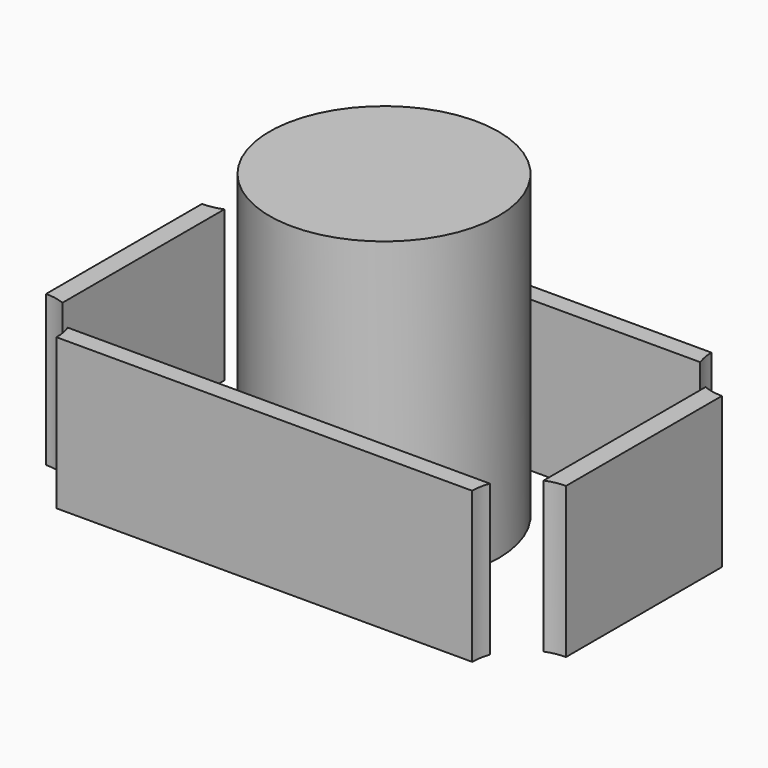
from build123d import *

# Parameters (mm, degrees)
F1_DEPTH = 25.4
F0_R     = 19.2971097636
F3_DEPTH = 50.8


# Not quite as in the source:
# - the program builds the solid bodies; features that only make, move or delete a surface that nothing else refers to are left out


with BuildPart() as f1:
    # F0 (on Top) → F1 (new body)
    with BuildSketch(Plane.XY):
        with BuildLine():
            Line((35.0388884567, 25.2227913588), (-35.0388884567, 25.2227913588))
            ThreePointArc((-35.0388884567, 25.2227913588), (-35.1771760377, 23.6696604158), (-35.5876880321, 22.1653934568))
            Line((-35.5876880321, 22.1653934568), (35.5876880321, 22.1653934568))
            ThreePointArc((35.5876880321, 22.1653934568), (35.1771760377, 23.6696604158), (35.0388884567, 25.2227913588))
        make_face()
    extrude(amount=F1_DEPTH)


with BuildPart() as f1b:
    # F0 (on Top) → F1, piece 2 (new body)
    with BuildSketch(Plane.XY):
        with BuildLine():
            Line((40.5652746558, 17.0605210708), (40.5652746558, -17.0605210708))
            ThreePointArc((40.5652746558, -17.0605210708), (42.1675359576, -16.590493834), (43.8297688961, -16.4319109195))
            Line((43.8297688961, -16.4319109195), (43.8297688961, 16.4319109195))
            ThreePointArc((43.8297688961, 16.4319109195), (42.1675359576, 16.590493834), (40.5652746558, 17.0605210708))
        make_face()
    extrude(amount=F1_DEPTH)


with BuildPart() as f1c:
    # F0 (on Top) → F1, piece 3 (new body)
    with BuildSketch(Plane.XY):
        with BuildLine():
            Line((-43.8297688961, 16.4319109195), (-43.8297688961, -16.4319109195))
            ThreePointArc((-43.8297688961, -16.4319109195), (-42.1675359576, -16.590493834), (-40.5652746558, -17.0605210708))
            Line((-40.5652746558, -17.0605210708), (-40.5652746558, 17.0605210708))
            ThreePointArc((-40.5652746558, 17.0605210708), (-42.1675359576, 16.590493834), (-43.8297688961, 16.4319109195))
        make_face()
    extrude(amount=F1_DEPTH)


with BuildPart() as f1d:
    # F0 (on Top) → F1, piece 4 (new body)
    with BuildSketch(Plane.XY):
        with BuildLine():
            Line((-35.0388884567, -25.2227913588), (35.0388884567, -25.2227913588))
            ThreePointArc((35.0388884567, -25.2227913588), (35.1771760377, -23.6696604158), (35.5876880321, -22.1653934568))
            Line((35.5876880321, -22.1653934568), (-35.5876880321, -22.1653934568))
            ThreePointArc((-35.5876880321, -22.1653934568), (-35.1771760377, -23.6696604158), (-35.0388884567, -25.2227913588))
        make_face()
    extrude(amount=F1_DEPTH)


with BuildPart() as f3:
    # F0 (on Top) → F3 (new body)
    with BuildSketch(Plane.XY):
        Circle(F0_R)
    extrude(amount=F3_DEPTH)


solid = Compound([f1.part, f1b.part, f1c.part, f1d.part, f3.part])
